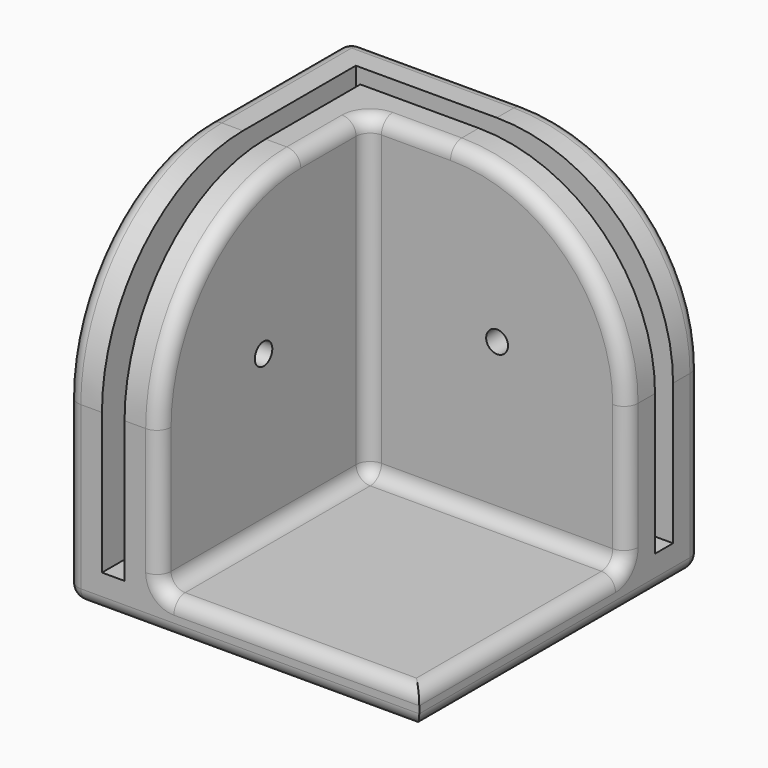
from build123d import *

# Parameters (mm, degrees)
F0_W            = 50
F0_H            = 50
F1_DEPTH        = 5
F2_W            = 45
F2_H            = 5
F3_DEPTH        = 45
F4_W            = 36.8
F4_H            = 5
F5_DEPTH        = 45
F6_R            = 25
F7_R            = 2
F10_D           = 3.1
F10_DEPTH       = 20
F10_TIP         = 0.9313339595
F10_ON_F9_D     = 3.1
F10_ON_F9_DEPTH = 20
F10_ON_F9_TIP   = 0.9313339595


with BuildPart() as f1:
    # F0 (on Top) → F1 (new body)
    with BuildSketch(Plane.XY):
        Rectangle(F0_W, F0_H)
    extrude(amount=F1_DEPTH)

    # F2 (on face) → F3 (join)
    with BuildSketch(Plane.XY.offset(5)):
        Polygon((-20, 25), (-25, 25), (-25, -25), (-20, -25), (-20, 20), align=None)
        with Locations((2.5, 22.5)):
            Rectangle(F2_W, F2_H)
    extrude(amount=F3_DEPTH)

    # F4 (on face) → F5 (join, through all)
    with BuildSketch(Plane.XY.offset(5)):
        Polygon((-16.8, 16.8), (-16.8, -25), (-11.8, -25), (-11.8, 11.8), (-11.8, 16.8), align=None)
        with Locations((6.6, 14.3)):
            Rectangle(F4_W, F4_H)
    extrude(amount=F5_DEPTH)

    # F6
    f6_edges = [f1.edges().sort_by_distance(p)[0] for p in [
        (-22.5, -25, 50),
        (-14.3, -25, 50),
        (25, 14.3, 50),
        (25, 22.5, 50),
    ]]
    fillet(f6_edges, radius=F6_R)

    # F7
    f7_edges = [f1.edges().sort_by_distance(p)[0] for p in [
        (25, 25, 12.5),
        (17.67767, 25, 42.67767),
        (0, 25, 0),
        (-12.5, 25, 50),
        (-25, 25, 25),
        (0, -25, 0),
        (25, 0, 0),
        (-25, 0, 0),
        (-25, 12.5, 50),
        (-25, -17.67767, 42.67767),
        (-25, -25, 12.5),
        (-11.8, -6.6, 5),
        (6.6, 11.8, 5),
        (25, -6.6, 5),
        (6.6, -25, 5),
        (-11.8, 11.8, 27.5),
        (-11.8, -25, 15),
        (25, 11.8, 15),
        (-11.8, -17.67767, 42.67767),
        (-11.8, 5.9, 50),
        (17.67767, 11.8, 42.67767),
        (-5.9, 11.8, 50),
    ]]
    fillet(f7_edges, radius=F7_R)

    # F10
    with Locations(Plane.YZ.offset(-11.8)):
        with Locations((-6.6, 27.5)):
            Hole(F10_D / 2, depth=F10_DEPTH)
            with Locations((0, 0, -(F10_DEPTH + F10_TIP / 2))):  # 118° drill point
                Cone(0, F10_D / 2, F10_TIP, mode=Mode.SUBTRACT)

    # F10 on F9
    with Locations(Plane.XZ.offset(-11.8)):
        with Locations((6.6, 27.5)):
            Hole(F10_ON_F9_D / 2, depth=F10_ON_F9_DEPTH)
            with Locations((0, 0, -(F10_ON_F9_DEPTH + F10_ON_F9_TIP / 2))):  # 118° drill point
                Cone(0, F10_ON_F9_D / 2, F10_ON_F9_TIP, mode=Mode.SUBTRACT)


solid = f1.part
